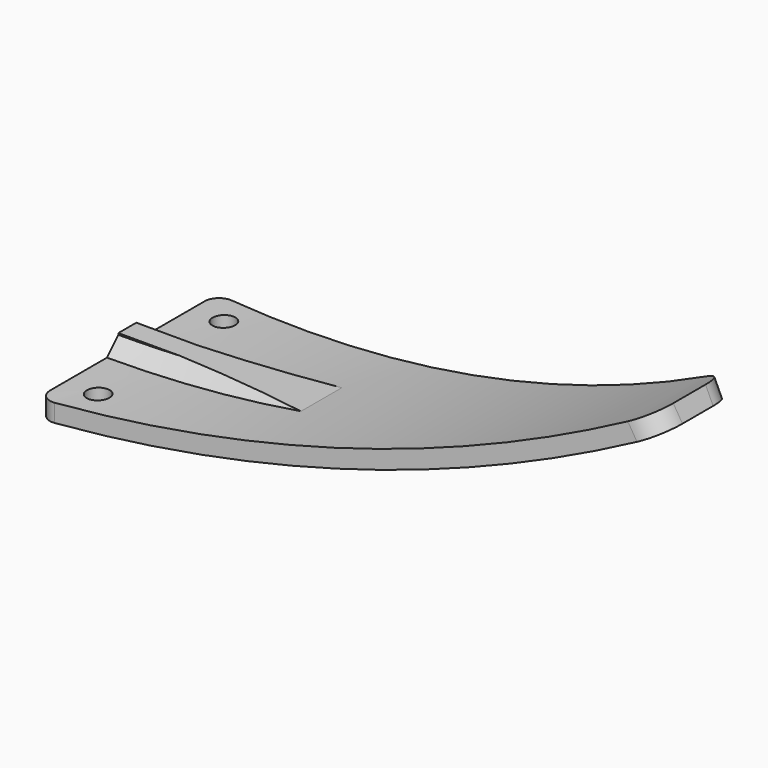
from build123d import *

# Parameters (mm, degrees)
F1_DEPTH      = 20
F1_DEPTH_BACK = 20
F2_R          = 2
F3_DEPTH      = 25.4
F5_DEPTH      = 50.8
F7_DEPTH      = 2
F7_DEPTH_BACK = 2
F8_SIZE       = 2.54
F9_R          = 5.08
F10_T1_DEPTH  = 15.875
F11_T1_DEPTH  = 18.9511481059


# Not quite as in the source:
# - a fillet or chamfer that OpenCascade refuses, or shapes differently, is made with other operations: its cross-section is extruded or revolved along the edge and cut away or added


with BuildPart() as f1:
    # F0 (on Front) → F1 (new body, two sides)
    with BuildSketch(Plane.XZ) as f1_sk:
        with BuildLine():
            Line((0, 3.175), (0, 0))
            ThreePointArc((0, 0), (52.3634414453, 6.4462342186), (101.6, 25.4))
            Line((101.6, 25.4), (100.1058823529, 28.2014705882))
            ThreePointArc((100.1058823529, 28.2014705882), (51.5933908359, 9.5264366566), (0, 3.175))
        make_face()
    extrude(amount=F1_DEPTH)
    extrude(f1_sk.sketch, amount=-F1_DEPTH_BACK)

    # F2 (on Top) → F3 (cut)
    with BuildSketch(Plane.XY):
        with Locations((6, 14)):
            Circle(F2_R)
        with Locations((6, -14)):
            Circle(F2_R)
    extrude(amount=F3_DEPTH, mode=Mode.SUBTRACT)

    # F4 (on Top) → F5 (cut)
    with BuildSketch(Plane.XY):
        Polygon((0.5, 20), (101.6, 8), (101.6, 20), align=None)
        Polygon((101.6, -8), (0.5, -20), (101.6, -20), align=None)
    extrude(amount=F5_DEPTH, mode=Mode.SUBTRACT)

    # F6 (on Front) → F7 (join, two sides)
    with BuildSketch(Plane.XZ) as f7_sk:
        Polygon((0, 6), (0, 0), (37, 6), align=None)
    extrude(amount=F7_DEPTH)
    extrude(f7_sk.sketch, amount=-F7_DEPTH_BACK)

    # F8
    f8_edges = [f1.edges().sort_by_distance(p)[0] for p in [
        (17.334188, -2, 3.882426),
        (17.334188, 2, 3.882426),
    ]]
    chamfer(f8_edges, length=F8_SIZE)

    # F9
    f9_edges = [f1.edges().sort_by_distance(p)[0] for p in [
        (100.852941, -8.088672, 26.800735),
        (100.852941, 8.088672, 26.800735),
    ]]
    fillet(f9_edges, radius=F9_R)

    # F10: fillet of radius 2.54 on 2 edges, made by hand

    # F10_s2 → F10_t1 (cut)
    with BuildSketch(Plane.XY.offset(-6.35)):
        with BuildLine():
            ThreePointArc((0, -17.46), (0.7439487758, -19.2560512242), (2.54, -20))
            Line((2.54, -20), (0, -20))
            Line((0, -20), (0, -17.46))
        make_face()
        with BuildLine():
            ThreePointArc((2.54, 20), (0.7439487758, 19.2560512242), (0, 17.46))
            Line((0, 17.46), (0, 20))
            Line((0, 20), (2.54, 20))
        make_face()
    extrude(amount=F10_T1_DEPTH, mode=Mode.SUBTRACT)

    # F11: fillet of radius 2.54 on 2 edges, made by hand

    # F11_s2 → F11_t1 (cut)
    with BuildSketch(Plane.XY.offset(-7.8813228745)):
        with BuildLine():
            ThreePointArc((0, -17.2000338729), (0.8531139151, -19.0989849877), (2.8393821549, -19.7223285276))
            Line((2.8393821549, -19.7223285276), (2.8693203704, -19.9745579931))
            Line((2.8693203704, -19.9745579931), (1.7309730402, -20.1096734032))
            Line((1.7309730402, -20.1096734032), (1.6171383071, -20.0971883315))
            ThreePointArc((1.6171383071, -20.0971883315), (-0.254, -17.46), (-0.254, -17.2000338729))
            Line((-0.254, -17.2000338729), (0, -17.2000338729))
        make_face()
        with BuildLine():
            ThreePointArc((0, 17.2000338729), (0.8531139151, 19.0989849877), (2.8393821549, 19.7223285276))
            Line((2.8393821549, 19.7223285276), (2.8693203704, 19.9745579931))
            Line((2.8693203704, 19.9745579931), (1.7309730402, 20.1096734032))
            Line((1.7309730402, 20.1096734032), (1.6171383071, 20.0971883315))
            ThreePointArc((1.6171383071, 20.0971883315), (-0.254, 17.46), (-0.254, 17.2000338729))
            Line((-0.254, 17.2000338729), (0, 17.2000338729))
        make_face()
    extrude(amount=F11_T1_DEPTH, mode=Mode.SUBTRACT)


solid = f1.part
